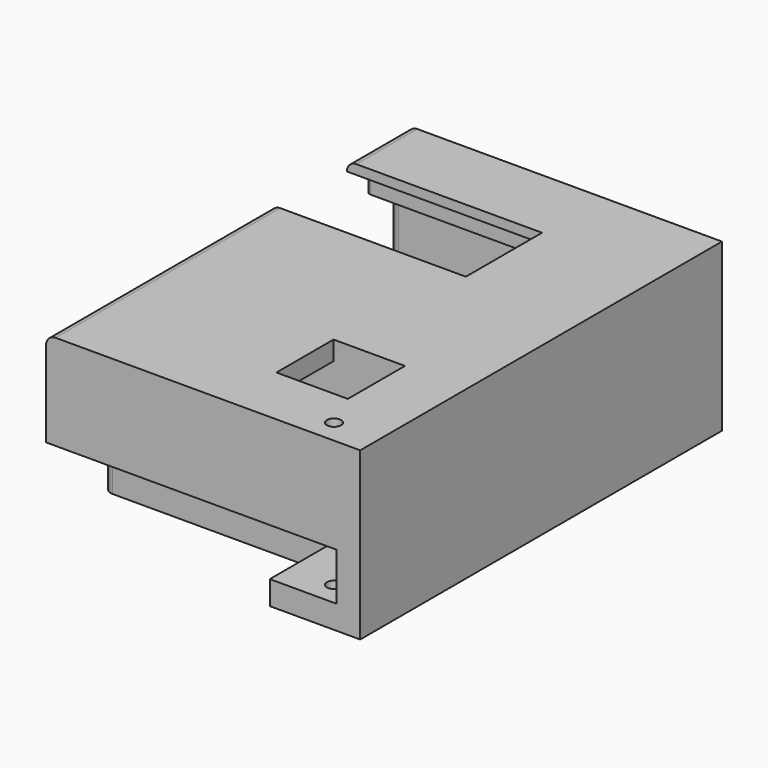
from build123d import *

# Parameters (mm, degrees)
F1_DEPTH     = 5
F3_DEPTH     = 30
F5_DEPTH     = 61
F6_W         = 41
F6_H         = 20
F6_W_2       = 15
F6_H_2       = 15
F7_DEPTH     = 4.001
F8_R         = 1.5
F9_DEPTH     = 35.001
F10_R        = 2
F11_T1_DEPTH = 8.5
F11_T3_DEPTH = 4
F11_T5_DEPTH = 59
F11_T8_ANGLE = 90


# Not quite as in the source:
# - a fillet or chamfer that OpenCascade refuses, or shapes differently, is made with other operations: its cross-section is extruded or revolved along the edge and cut away or added


with BuildPart() as f1:
    # F0 (on Top) → F1 (new body)
    with BuildSketch(Plane.XY):
        Polygon((33, 47.5), (-33, 47.5), (-33, -32.5), (14, -32.5), (14, -47.5), (33, -47.5), align=None)
    extrude(amount=F1_DEPTH)

    # F2 (on face) → F3 (join)
    with BuildSketch(Plane.XY.offset(5)):
        Polygon((-33, 42.5), (28, 42.5), (28, -47.5), (33, -47.5), (33, 47.5), (-33, 47.5), align=None)
    extrude(amount=F3_DEPTH)

    # F4 (on face) → F5 (join, through all)
    with BuildSketch(Plane(origin=(28, 0, 0), x_dir=(0, -1, 0), z_dir=(-1, 0, 0))):
        Polygon((47.5, 35), (-42.5, 35), (-42.5, 27), (-36.5, 27), (-36.5, 33), (-6.5, 33), (-6.5, 27), (8.5, 27), (8.5, 15), (19.5, 15), (19.5, 31), (37.5, 31), (37.5, 15), (47.5, 15), align=None)
    extrude(amount=F5_DEPTH)

    # F6 (on face) → F7 (cut, through all)
    with BuildSketch(Plane.XY.offset(35)):
        with Locations((-12.5, 21.5)):
            Rectangle(F6_W, F6_H)
        with Locations((12.5, -27)):
            Rectangle(F6_W_2, F6_H_2)
    extrude(amount=-F7_DEPTH, mode=Mode.SUBTRACT)

    # F8 (on face) → F9 (cut, through all)
    with BuildSketch(Plane(origin=(0, 0, 0), x_dir=(1, 0, 0), z_dir=(0, 0, -1))):
        with Locations((23.5, 42.5)):
            Circle(F8_R)
    extrude(amount=-F9_DEPTH, mode=Mode.SUBTRACT)

    # F10
    f10_edges = [f1.edges().sort_by_distance(p)[0] for p in [
        (-33, -18, 35),
        (-33, 39.5, 35),
        (-33, -19.5, 23),
        (-33, -37.5, 23),
        (-33, -8.5, 21),
        (-33, -1, 27),
        (-33, 42.5, 16),
        (-33, -32.5, 2.5),
    ]]
    fillet(f10_edges, radius=F10_R)

    # F11: fillet of radius 1 on 2 edges, made by hand

    # F11_s2 → F11_t1 (cut)
    with BuildSketch(Plane.XY.offset(24.5)):
        with BuildLine():
            ThreePointArc((-33, 37.5), (-32.7071067812, 36.7928932188), (-32, 36.5))
            Line((-32, 36.5), (-33, 36.5))
            Line((-33, 36.5), (-33, 37.5))
        make_face()
    extrude(amount=F11_T1_DEPTH, mode=Mode.SUBTRACT)

    # F11_s4 → F11_t3 (cut)
    with BuildSketch(Plane.XY.offset(29)):
        with BuildLine():
            ThreePointArc((-33, 5.5), (-32.7071067812, 6.2071067812), (-32, 6.5))
            Line((-32, 6.5), (-33, 6.5))
            Line((-33, 6.5), (-33, 5.5))
        make_face()
    extrude(amount=F11_T3_DEPTH, mode=Mode.SUBTRACT)

    # F11_s6 → F11_t5 (cut)
    with BuildSketch(Plane.YZ.offset(-31)):
        with BuildLine():
            ThreePointArc((6.5, 28), (6.2071067812, 27.2928932188), (5.5, 27))
            Line((5.5, 27), (6.5, 27))
            Line((6.5, 27), (6.5, 28))
        make_face()
    extrude(amount=F11_T5_DEPTH, mode=Mode.SUBTRACT)

    # F11_s7 → F11_t8 (revolve, cut)
    with BuildSketch(Plane.XY.offset(29)):
        with BuildLine():
            ThreePointArc((-32, 6.5), (-32.7071067812, 6.2071067812), (-33, 5.5))
            Line((-33, 5.5), (-33, 6.5))
            Line((-33, 6.5), (-32, 6.5))
        make_face()
    revolve(axis=Axis((-31, 6.5, 29), (0, -1, 0)), revolution_arc=F11_T8_ANGLE, mode=Mode.SUBTRACT)


solid = f1.part
